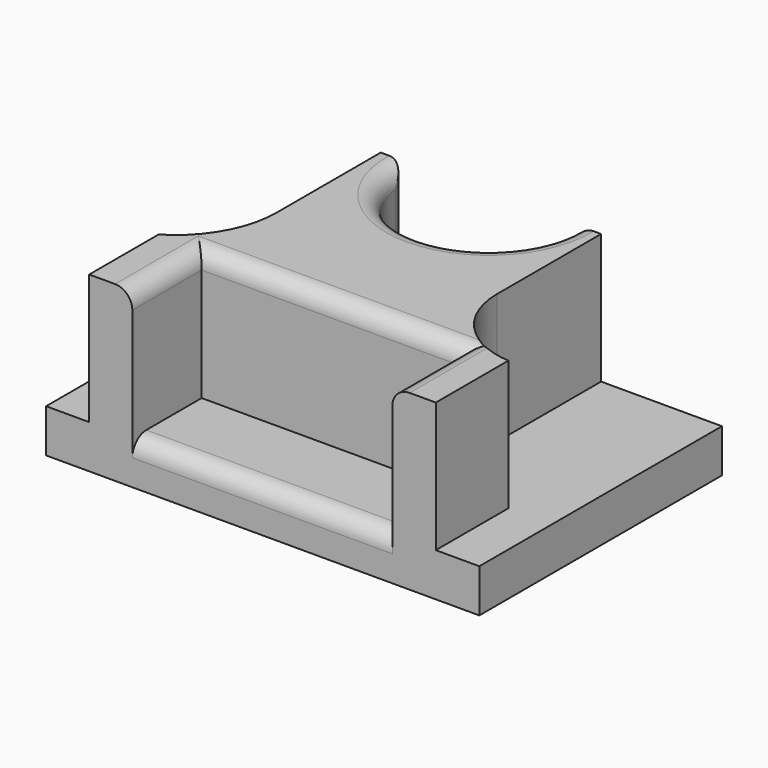
from build123d import *

# Parameters (mm, degrees)
F0_W         = 127
F0_H         = 88.9
F1_DEPTH     = 50.8
F3_DEPTH     = 76.2
F4_W         = 76.2
F4_H         = 25.4
F5_DEPTH     = 38.1
F7_DEPTH     = 38.1
F8_T1_DEPTH  = 76.2
F8_T3_DEPTH  = 38.1
F8_T5_DEPTH  = 74.8723933942
F8_T8_ANGLE  = 242.9501193557
F8_T10_ANGLE = 242.9501193557
F8_T15_DEPTH = 38.1
F8_S16_R     = 24.2542650998
F8_T17_DEPTH = 21
F8_T21_DEPTH = 88.9
F8_S22_R     = 24.2542650998
F8_T23_DEPTH = 46
F8_T30_DEPTH = 88.9
F8_S32_R     = 29.6655396369
F8_T33_DEPTH = 46
F8_T36_DEPTH = 38.1
F8_S38_R     = 29.6655396369
F8_T39_DEPTH = 21


# Not quite as in the source:
# - a fillet or chamfer that OpenCascade refuses, or shapes differently, is made with other operations: its cross-section is extruded or revolved along the edge and cut away or added


with BuildPart() as f1:
    # F0 (on Top) → F1 (new body)
    with BuildSketch(Plane.XY):
        with Locations((0.947636019, -9.969078747)):
            Rectangle(F0_W, F0_H)
    extrude(amount=F1_DEPTH)

    # F2 (on face) → F3 (cut)
    with BuildSketch(Plane.XY.offset(50.8)):
        with BuildLine():
            Line((21.7591244727, 34.480921253), (-28.0215628445, 34.480921253))
            ThreePointArc((-28.0215628445, 34.480921253), (-3.1312191859, 8.6101276845), (21.7591244727, 34.480921253))
        make_face()
    extrude(amount=-F3_DEPTH, mode=Mode.SUBTRACT)

    # F4 (on face) → F5 (cut)
    with BuildSketch(Plane.XY.offset(50.8)):
        with Locations((0.8347104251, -41.719078747)):
            Rectangle(F4_W, F4_H)
    extrude(amount=-F5_DEPTH, mode=Mode.SUBTRACT)

    # F6 (on face) → F7 (cut)
    with BuildSketch(Plane.XY.offset(50.8)):
        with BuildLine():
            Line((-62.552363981, -54.419078747), (-49.9088267779, -54.419078747))
            Line((-49.9088267779, -54.419078747), (-49.9088267779, -29.019078747))
            ThreePointArc((-49.9088267779, -29.019078747), (-39.401677619, -18.2031822516), (-35.5692207813, -3.619078747))
            Line((-35.5692207813, -3.619078747), (-35.5692207813, 34.480921253))
            Line((-35.5692207813, 34.480921253), (-62.552363981, 34.480921253))
            Line((-62.552363981, 34.480921253), (-62.552363981, -54.419078747))
        make_face()
        with BuildLine():
            Line((51.6911732221, -27.8206840158), (51.6911732221, -54.419078747))
            Line((51.6911732221, -54.419078747), (64.447636019, -54.419078747))
            Line((64.447636019, -54.419078747), (64.447636019, 34.480921253))
            Line((64.447636019, 34.480921253), (29.0343053639, 34.480921253))
            Line((29.0343053639, 34.480921253), (29.0343053639, -3.619078747))
            ThreePointArc((29.0343053639, -3.619078747), (35.5824546884, -20.1950505038), (51.6911732221, -27.8206840158))
        make_face()
    extrude(amount=-F7_DEPTH, mode=Mode.SUBTRACT)

    # F8: fillet of radius 5.08 on 8 edges, made by hand

    # F8_s2 → F8_t1 (cut)
    with BuildSketch(Plane.YZ.offset(-37.2652895749)):
        with BuildLine():
            ThreePointArc((-23.939078747, 50.8), (-27.5311811954, 49.3121024484), (-29.019078747, 45.72))
            Line((-29.019078747, 45.72), (-29.019078747, 50.8))
            Line((-29.019078747, 50.8), (-23.939078747, 50.8))
        make_face()
        with BuildLine():
            ThreePointArc((-54.419078747, 7.62), (-52.9311811954, 11.2121024484), (-49.339078747, 12.7))
            Line((-49.339078747, 12.7), (-54.419078747, 12.7))
            Line((-54.419078747, 12.7), (-54.419078747, 7.62))
        make_face()
    extrude(amount=F8_T1_DEPTH, mode=Mode.SUBTRACT)

    # F8_s4 → F8_t3 (cut)
    with BuildSketch(Plane.XZ.offset(29.019078747)):
        with BuildLine():
            ThreePointArc((-42.3452895749, 50.8), (-38.7531871264, 49.3121024484), (-37.2652895749, 45.72))
            Line((-37.2652895749, 45.72), (-37.2652895749, 50.8))
            Line((-37.2652895749, 50.8), (-42.3452895749, 50.8))
        make_face()
        with BuildLine():
            ThreePointArc((44.0147104251, 50.8), (40.4226079767, 49.3121024484), (38.9347104251, 45.72))
            Line((38.9347104251, 45.72), (38.9347104251, 50.8))
            Line((38.9347104251, 50.8), (44.0147104251, 50.8))
        make_face()
    extrude(amount=F8_T3_DEPTH, mode=Mode.SUBTRACT)

    # F8_s6 → F8_t5 (cut)
    with BuildSketch(Plane.XY.offset(-12.0361966971)):
        with BuildLine():
            ThreePointArc((26.5736031516, 34.480921253), (23.2372411895, 33.2317291127), (21.5417284952, 30.0985152915))
            ThreePointArc((21.5417284952, 30.0985152915), (21.7471113974, 32.2849220687), (21.7591244727, 34.480921253))
            Line((21.7591244727, 34.480921253), (26.5736031516, 34.480921253))
        make_face()
        with BuildLine():
            ThreePointArc((-32.8360415234, 34.480921253), (-29.4996795612, 33.2317291127), (-27.804166867, 30.0985152915))
            ThreePointArc((-27.804166867, 30.0985152915), (-28.0095497691, 32.2849220687), (-28.0215628445, 34.480921253))
            Line((-28.0215628445, 34.480921253), (-32.8360415234, 34.480921253))
        make_face()
    extrude(amount=F8_T5_DEPTH, mode=Mode.SUBTRACT)

    # F8_s7 → F8_t8 (revolve, cut)
    with BuildSketch(Plane(origin=(14.0725928873, 22.9868383553, 0), x_dir=(0, 0, 1), z_dir=(0.5221273689, 0.8528675224, 0))):
        with BuildLine():
            ThreePointArc((45.72, -45.0806506369), (49.3121024484, -46.5685481884), (50.8, -50.1606506369))
            Line((50.8, -50.1606506369), (50.8, -45.0806506369))
            Line((50.8, -45.0806506369), (45.72, -45.0806506369))
        make_face()
    revolve(axis=Axis((-3.1312191859, 33.5190498615, 50.8), (0, 0, 1)), revolution_arc=F8_T8_ANGLE, mode=Mode.SUBTRACT)

    # F8_s9 → F8_t10 (revolve, cut)
    with BuildSketch(Plane(origin=(14.0725928873, 22.9868383553, 0), x_dir=(0, 0, 1), z_dir=(0.5221273689, 0.8528675224, 0))):
        with BuildLine():
            ThreePointArc((0, -50.1606506369), (1.4878975516, -46.5685481884), (5.08, -45.0806506369))
            Line((5.08, -45.0806506369), (0, -45.0806506369))
            Line((0, -45.0806506369), (0, -50.1606506369))
        make_face()
    revolve(axis=Axis((-3.1312191859, 33.5190498615, 0), (0, 0, 1)), revolution_arc=F8_T10_ANGLE, mode=Mode.SUBTRACT)


with BuildPart() as f8_tool13:
    # F8_s14 → F8_t15 (new body)
    with BuildSketch(Plane.XZ.offset(54.419078747)):
        with BuildLine():
            ThreePointArc((44.0147104251, 50.8), (40.4226079767, 49.3121024484), (38.9347104251, 45.72))
            Line((38.9347104251, 45.72), (38.9347104251, 50.8))
            Line((38.9347104251, 50.8), (44.0147104251, 50.8))
        make_face()
    extrude(amount=-F8_T15_DEPTH)

    # F8_s16 → F8_t17 (cut, symmetric)
    with BuildSketch(Plane.XY.offset(48.3)):
        with Locations((53.2885704637, -3.619078747)):
            Circle(F8_S16_R)
    extrude(amount=F8_T17_DEPTH, both=True, mode=Mode.SUBTRACT)

    split(bisect_by=Plane.XZ.offset(29.019078747), keep=Keep.BOTTOM)


with BuildPart() as f8_tool19:
    # F8_s20 → F8_t21 (new body)
    with BuildSketch(Plane.YZ.offset(51.6347104251)):
        with BuildLine():
            ThreePointArc((-23.939078747, 50.8), (-27.5311811954, 49.3121024484), (-29.019078747, 45.72))
            Line((-29.019078747, 45.72), (-29.019078747, 50.8))
            Line((-29.019078747, 50.8), (-23.939078747, 50.8))
        make_face()
    extrude(amount=-F8_T21_DEPTH)

    # F8_s22 → F8_t23 (cut, symmetric)
    with BuildSketch(Plane.XY.offset(48.3)):
        with Locations((53.2885704637, -3.619078747)):
            Circle(F8_S22_R)
    extrude(amount=F8_T23_DEPTH, both=True, mode=Mode.SUBTRACT)

    split(bisect_by=Plane.YZ.offset(38.9347104251), keep=Keep.TOP)


with BuildPart() as f8_tool13_1:
    add(f8_tool13.part)

    # F8_t25: intersect F8_tool19
    add(f8_tool19.part, mode=Mode.INTERSECT)


with BuildPart() as f1_1:
    add(f1.part)

    # F8_t11: cut F8_tool13
    add(f8_tool13_1.part, mode=Mode.SUBTRACT)


with BuildPart() as f8_tool28:
    # F8_s29 → F8_t30 (new body)
    with BuildSketch(Plane.YZ.offset(38.9347104251)):
        with BuildLine():
            ThreePointArc((-23.939078747, 50.8), (-27.5311811954, 49.3121024484), (-29.019078747, 45.72))
            Line((-29.019078747, 45.72), (-29.019078747, 50.8))
            Line((-29.019078747, 50.8), (-23.939078747, 50.8))
        make_face()
    extrude(amount=-F8_T30_DEPTH)

    split(bisect_by=Plane.YZ.offset(-37.2652895749), keep=Keep.BOTTOM)

    # F8_s32 → F8_t33 (cut, symmetric)
    with BuildSketch(Plane.XY.offset(48.3)):
        with Locations((-65.2347604182, -3.619078747)):
            Circle(F8_S32_R)
    extrude(amount=F8_T33_DEPTH, both=True, mode=Mode.SUBTRACT)


with BuildPart() as f8_tool34:
    # F8_s35 → F8_t36 (new body)
    with BuildSketch(Plane.XZ.offset(16.319078747)):
        with BuildLine():
            ThreePointArc((-42.3452895749, 50.8), (-38.7531871264, 49.3121024484), (-37.2652895749, 45.72))
            Line((-37.2652895749, 45.72), (-37.2652895749, 50.8))
            Line((-37.2652895749, 50.8), (-42.3452895749, 50.8))
        make_face()
    extrude(amount=F8_T36_DEPTH)

    split(bisect_by=Plane.XZ.offset(29.019078747), keep=Keep.BOTTOM)

    # F8_s38 → F8_t39 (cut, symmetric)
    with BuildSketch(Plane.XY.offset(48.3)):
        with Locations((-65.2347604182, -3.619078747)):
            Circle(F8_S38_R)
    extrude(amount=F8_T39_DEPTH, both=True, mode=Mode.SUBTRACT)


with BuildPart() as f8_tool28_1:
    add(f8_tool28.part)

    # F8_t40: intersect F8_tool34
    add(f8_tool34.part, mode=Mode.INTERSECT)


with BuildPart() as f1_2:
    add(f1_1.part)

    # F8_t26: cut F8_tool28
    add(f8_tool28_1.part, mode=Mode.SUBTRACT)


solid = f1_2.part
